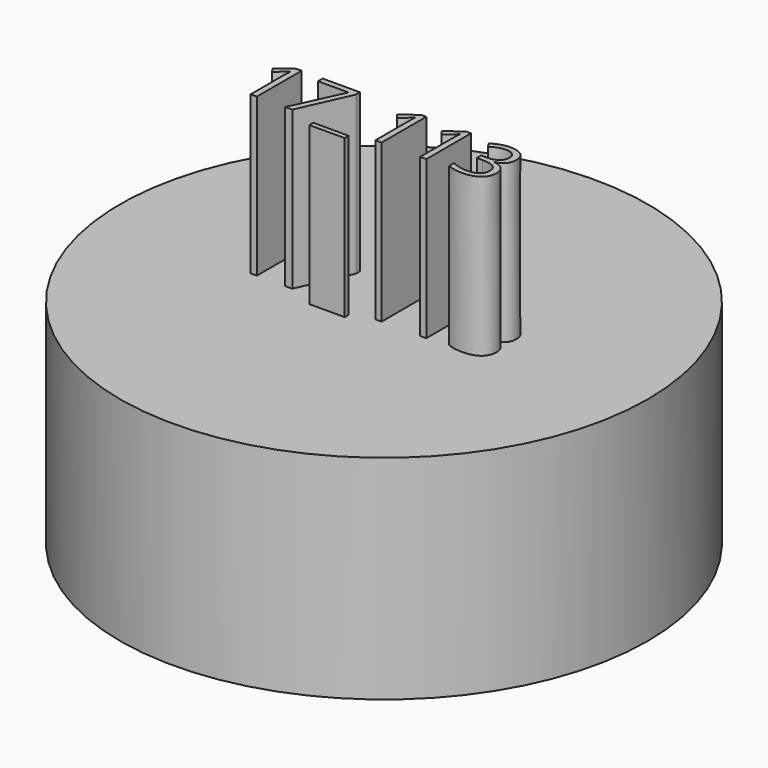
from build123d import *

# Parameters (mm, degrees)
F0_R         = 42.5259434293
F1_DEPTH     = 34.29
F2_TEXT_SIZE = 12.6175388383
F3_DEPTH     = 25.4


# Not quite as in the source:
# - Text() gives the source's letters only with a copy of the font that has no kerning and outlines rounded to 1/6400 em; it was checked with that copy


with BuildPart() as f1:
    # F0 (on Top) → F1 (new body)
    with BuildSketch(Plane.XY):
        Circle(F0_R)
    extrude(amount=F1_DEPTH)


with BuildPart() as f3:
    # F2 (on face) → F3 (new body)
    with BuildSketch(Plane.XY.offset(34.29)):
        with Locations((-21.328272298, -4.4347438961)):
            Text('17_113', F2_TEXT_SIZE, font='Open Sans', text_align=(TextAlign.LEFT, TextAlign.BOTTOM))
    extrude(amount=F3_DEPTH)


solid = Compound([f1.part, f3.part])
